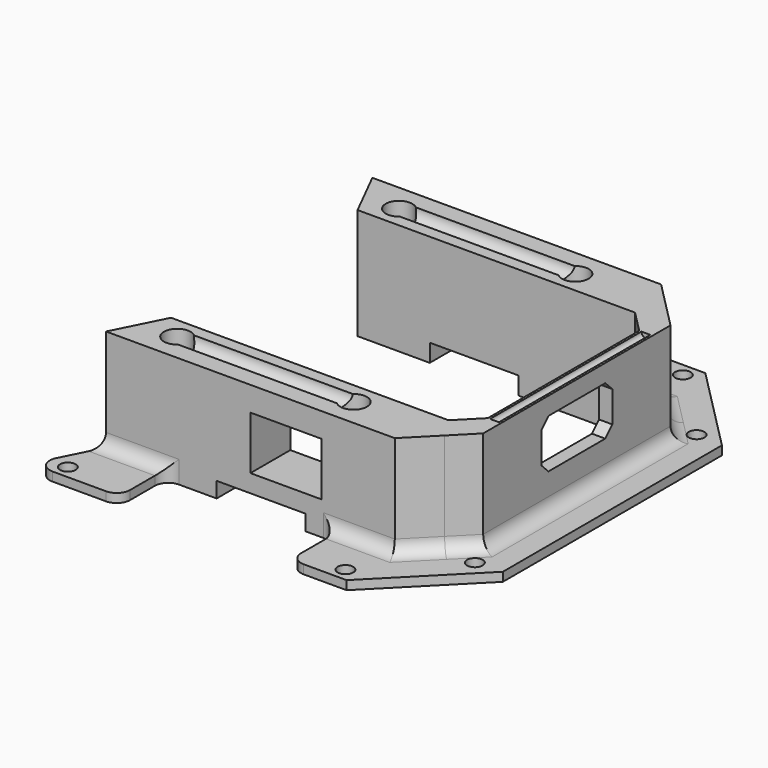
from build123d import *

# Parameters (mm, degrees)
F0_R      = 1.75
F1_DEPTH  = 2
F2_DEPTH  = 25
F3_W      = 10
F3_H      = 11
F4_DEPTH  = 12.5
F5_W      = 16
F5_H      = 12
F5_W_2    = 9.587623179
F5_H_2    = 49.3407100439
F5_W_3    = 20
F5_H_3    = 3.5
F6_W      = 20
F6_H      = 4
F7_DEPTH  = 12.5
F8_R      = 3
F10_DEPTH = 7.5
F11_W     = 1
F11_H     = 42.6
F15_SIZE  = 2


# Not quite as in the source:
# - a feature names something its author has since deleted; it is built from what else it names


with BuildPart() as f1:
    # F0 (on Top) → F1 (new body)
    with BuildSketch(Plane.XY):
        Polygon((-15.5396774872, 50.4744988004), (-9.0115841546, 37.4744988004), (4.3894230769, 37.4744988004), (4.3894230769, 50.4744988004), align=None)
        with Locations((-9.6105769231, 47.4744988004)):
            Circle(F0_R, mode=Mode.SUBTRACT)
    extrude(amount=F1_DEPTH)



with BuildPart() as f1b:
    # F0 (on Top) → F1, piece 2 (new body)
    with BuildSketch(Plane.XY):
        Polygon((55.9884158454, 37.4744988004), (62.1997159179, 31.2), (67, 26.3508739936), (67, -26.3508739936), (62.1997159179, -31.2), (55.9884158454, -37.4744988004), (42.8894230769, -37.4744988004), (42.8894230769, -50.4744988004), (55.5480775622, -50.4744988004), (75, -30.8246569672), (75, 30.8246569672), (55.5480775622, 50.4744988004), (42.8894230769, 50.4744988004), (42.8894230769, 37.4744988004), align=None)
        with Locations((52.8894230769, -47.4744988004)):
            Circle(F0_R, mode=Mode.SUBTRACT)
        with Locations((69, -31.2)):
            Circle(F0_R, mode=Mode.SUBTRACT)
        with Locations((69, 31.2)):
            Circle(F0_R, mode=Mode.SUBTRACT)
        with Locations((52.8894230769, 47.4744988004)):
            Circle(F0_R, mode=Mode.SUBTRACT)
    extrude(amount=F1_DEPTH)


with BuildPart() as f1c:
    # F0 (on Top) → F1, piece 3 (new body)
    with BuildSketch(Plane.XY):
        Polygon((4.3894230769, -50.4744988004), (4.3894230769, -37.4744988004), (-9.0115841546, -37.4744988004), (-15.5396774872, -50.4744988004), align=None)
        with Locations((-9.6105769231, -47.4744988004)):
            Circle(F0_R, mode=Mode.SUBTRACT)
    extrude(amount=F1_DEPTH)


with BuildPart() as f1_1:
    add(f1.part)

    add(f1b.part)  # F2 merges F1b

    add(f1c.part)  # F2 merges F1c
    # F0 (on Top) → F2 (join)
    with BuildSketch(Plane.XY):
        with BuildLine():
            ThreePointArc((-1, 31.2), (2, 34.2), (5, 31.2))
            Line((5, 31.2), (38.7, 31.2))
            ThreePointArc((38.7, 31.2), (41.7, 34.2), (44.7, 31.2))
            Line((44.7, 31.2), (54.1997159179, 31.2))
            Line((54.1997159179, 31.2), (62.1997159179, 31.2))
            Line((62.1997159179, 31.2), (55.9884158454, 37.4744988004))
            Line((55.9884158454, 37.4744988004), (42.8894230769, 37.4744988004))
            Line((42.8894230769, 37.4744988004), (4.3894230769, 37.4744988004))
            Line((4.3894230769, 37.4744988004), (-9.0115841546, 37.4744988004))
            Line((-9.0115841546, 37.4744988004), (-5.9652768733, 31.4081035087))
            Line((-5.9652768733, 31.4081035087), (-5.8607754019, 31.2))
            Line((-5.8607754019, 31.2), (-1, 31.2))
        make_face()
        with BuildLine():
            Line((55.9884158454, -37.4744988004), (62.1997159179, -31.2))
            Line((62.1997159179, -31.2), (54.1997159179, -31.2))
            Line((54.1997159179, -31.2), (44.7, -31.2))
            ThreePointArc((44.7, -31.2), (41.7, -34.2), (38.7, -31.2))
            Line((38.7, -31.2), (5, -31.2))
            ThreePointArc((5, -31.2), (2, -34.2), (-1, -31.2))
            Line((-1, -31.2), (-5.8607754019, -31.2))
            Line((-5.8607754019, -31.2), (-5.9652768733, -31.4081035087))
            Line((-5.9652768733, -31.4081035087), (-9.0115841546, -37.4744988004))
            Line((-9.0115841546, -37.4744988004), (4.3894230769, -37.4744988004))
            Line((4.3894230769, -37.4744988004), (42.8894230769, -37.4744988004))
            Line((42.8894230769, -37.4744988004), (55.9884158454, -37.4744988004))
        make_face()
        Polygon((62.1997159179, 31.2), (54.1997159179, 31.2), (59.0998579589, 26.25), (64, 21.3), (64, -21.3), (59.0998579589, -26.25), (54.1997159179, -31.2), (62.1997159179, -31.2), (67, -26.3508739936), (67, 26.3508739936), align=None)
        with BuildLine():
            Line((38.7, 31.2), (5, 31.2))
            ThreePointArc((5, 31.2), (2, 28.2), (-1, 31.2))
            Line((-1, 31.2), (-5.8607754019, 31.2))
            Line((-5.8607754019, 31.2), (-3.3750783253, 26.25))
            Line((-3.3750783253, 26.25), (59.0998579589, 26.25))
            Line((59.0998579589, 26.25), (54.1997159179, 31.2))
            Line((54.1997159179, 31.2), (44.7, 31.2))
            ThreePointArc((44.7, 31.2), (41.7, 28.2), (38.7, 31.2))
        make_face()
        with BuildLine():
            Line((54.1997159179, -31.2), (59.0998579589, -26.25))
            Line((59.0998579589, -26.25), (-3.3750783253, -26.25))
            Line((-3.3750783253, -26.25), (-5.8607754019, -31.2))
            Line((-5.8607754019, -31.2), (-1, -31.2))
            ThreePointArc((-1, -31.2), (2, -28.2), (5, -31.2))
            Line((5, -31.2), (38.7, -31.2))
            ThreePointArc((38.7, -31.2), (41.7, -28.2), (44.7, -31.2))
            Line((44.7, -31.2), (54.1997159179, -31.2))
        make_face()
    extrude(amount=F2_DEPTH)

    # F3 (on face) → F4 (cut, symmetric)
    with BuildSketch(Plane.YZ.offset(67)):
        with Locations((-5, 15.5)):
            Rectangle(F3_W, F3_H)
        with Locations((5, 15.5)):
            Rectangle(F3_W, F3_H)
    extrude(amount=F4_DEPTH, both=True, mode=Mode.SUBTRACT)

    # F5 (on face) + F6 (on face) → F7 (cut, symmetric)
    with BuildSketch(Plane.XZ.offset(37.4744988004)):
        with Locations((31.4884158454, 13.5)):
            Rectangle(F5_W, F5_H)
        with Locations((88.4978957474, 268.2395651937)):
            Rectangle(F5_W_2, F5_H_2)
        with Locations((25.8894230769, 1.75)):
            Rectangle(F5_W_3, F5_H_3)
    with BuildSketch(Plane(origin=(0, 37.4744988004, 0), x_dir=(-1, 0, 0), z_dir=(0, 1, 0))):
        with Locations((-22.8894230769, 2)):
            Rectangle(F6_W, F6_H)
    extrude(amount=F7_DEPTH, both=True, dir=(0, -1, 0), mode=Mode.SUBTRACT)

    # F8
    f8_edges = [f1_1.edges().sort_by_distance(p)[0] for p in [
        (49.438919, 37.474499, 2),
        (-2.311081, 37.474499, 2),
        (61.494208, 31.912686, 2),
        (67, 0, 2),
        (61.494208, -31.912686, 2),
        (49.438919, -37.474499, 2),
        (-2.311081, -37.474499, 2),
        (4.389423, 37.474499, 1),
        (42.889423, 37.474499, 1),
        (4.389423, -37.474499, 1),
        (42.889423, -37.474499, 1),
        (-15.539677, 50.474499, 1),
        (-15.539677, -50.474499, 1),
        (42.889423, 50.474499, 1),
        (4.389423, 50.474499, 1),
        (42.889423, -50.474499, 1),
        (4.389423, -50.474499, 1),
    ]]
    fillet(f8_edges, radius=F8_R)

    # F9 (on face) → F10 (cut)
    with BuildSketch(Plane(origin=(0, 0, 0), x_dir=(1, 0, 0), z_dir=(0, 0, -1))):
        with BuildLine():
            ThreePointArc((51.35, 31.2), (55.35, 27.2), (59.35, 31.2))
            ThreePointArc((59.35, 31.2), (55.35, 35.2), (51.35, 31.2))
        make_face()
        with BuildLine():
            Line((59.35, 26.25), (59.35, 31.2))
            ThreePointArc((59.35, 31.2), (55.35, 27.2), (51.35, 31.2))
            Line((51.35, 31.2), (51.35, 26.25))
            Line((51.35, 26.25), (59.0998579589, 26.25))
            Line((59.0998579589, 26.25), (59.35, 26.25))
        make_face()
        Polygon((59.35, 25.997312814), (59.35, 26.25), (59.0998579589, 26.25), align=None)
        with BuildLine():
            ThreePointArc((51.35, -31.2), (55.35, -35.2), (59.35, -31.2))
            ThreePointArc((59.35, -31.2), (55.35, -27.2), (51.35, -31.2))
        make_face()
        with BuildLine():
            ThreePointArc((51.35, -31.2), (55.35, -27.2), (59.35, -31.2))
            Line((59.35, -31.2), (59.35, -26.25))
            Line((59.35, -26.25), (59.0998579589, -26.25))
            Line((59.0998579589, -26.25), (51.35, -26.25))
            Line((51.35, -26.25), (51.35, -31.2))
        make_face()
        Polygon((59.0998579589, -26.25), (59.35, -26.25), (59.35, -25.997312814), align=None)
    extrude(amount=-F10_DEPTH, mode=Mode.SUBTRACT)

    # F11 (on face) → F12 (revolve, cut)
    with BuildSketch(Plane.XY.offset(25)):
        with Locations((66, 0)):
            Rectangle(F11_W, F11_H)
    revolve(axis=Axis((65.5, 0, 25), (0, -1, 0)), mode=Mode.SUBTRACT)

    # F11 (on face) → F13 (revolve, cut)
    with BuildSketch(Plane.XY.offset(25)):
        with BuildLine():
            ThreePointArc((3.9843134833, 33.45), (4.7343134833, 32.4343134833), (5, 31.2))
            Line((5, 31.2), (38.7, 31.2))
            ThreePointArc((38.7, 31.2), (38.9656865167, 32.4343134833), (39.7156865167, 33.45))
            Line((39.7156865167, 33.45), (3.9843134833, 33.45))
        make_face()
    revolve(axis=Axis((21.85, 31.2, 25), (1, 0, 0)), mode=Mode.SUBTRACT)

    # F11 (on face) → F14 (revolve, cut)
    with BuildSketch(Plane.XY.offset(25)):
        with BuildLine():
            Line((5, -31.2), (38.7, -31.2))
            ThreePointArc((38.7, -31.2), (38.9656865167, -29.9656865167), (39.7156865167, -28.95))
            Line((39.7156865167, -28.95), (3.9843134833, -28.95))
            ThreePointArc((3.9843134833, -28.95), (4.7343134833, -29.9656865167), (5, -31.2))
        make_face()
    revolve(axis=Axis((21.85, -31.2, 25), (1, 0, 0)), mode=Mode.SUBTRACT)

    # F15
    f15_edges = [f1_1.edges().sort_by_distance(p)[0] for p in [
        (65.5, -10, 21),
        (65.5, 10, 21),
        (65.5, -10, 10),
        (65.5, 10, 10),
    ]]
    chamfer(f15_edges, length=F15_SIZE)


solid = f1_1.part
